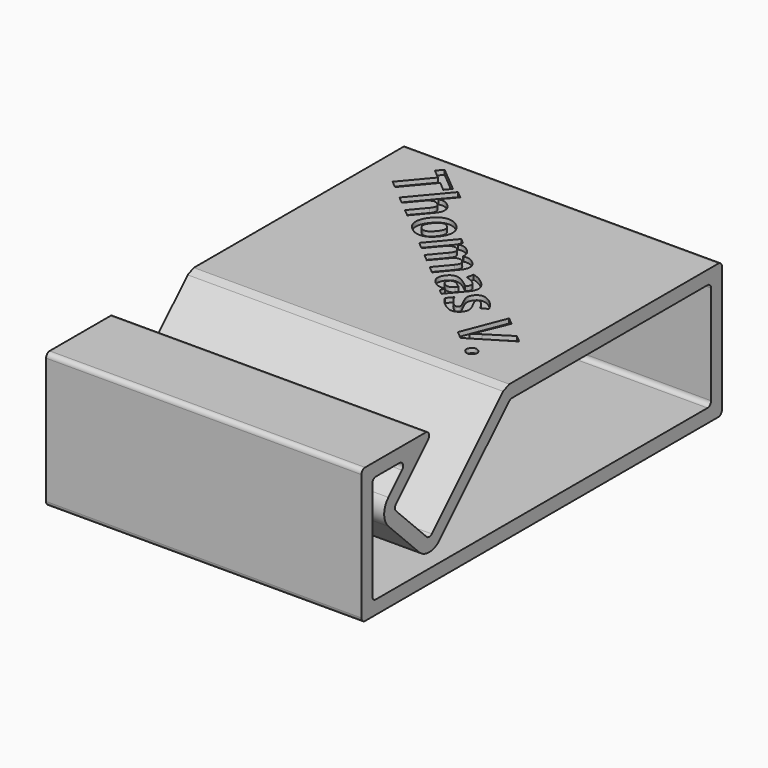
from build123d import *

# Parameters (mm, degrees)
F0_W         = 70
F0_H         = 100
F1_DEPTH     = 30
F3_DEPTH     = 146
F4_R         = 1
F5_SIZE      = 1
F6_T         = -3
F7_TEXT_SIZE = 13.6161935445
F8_DEPTH     = 1
F9_R         = 1
F10_R        = 1


# Not quite as in the source:
# - Text() gives the source's letters only with a copy of the font that has no kerning and outlines rounded to 1/6400 em; it was checked with that copy


with BuildPart() as f1:
    # F0 (on Top) → F1 (new body)
    with BuildSketch(Plane.XY):
        Rectangle(F0_W, F0_H)
    extrude(amount=F1_DEPTH)

    # F2 (on face) → F3 (cut)
    with BuildSketch(Plane.YZ.offset(35)):
        Polygon((-31.2132034356, 8.7867965644), (-10, 30), (-29.7989898732, 30), (-41.1126983722, 18.686291501), align=None)
    extrude(amount=-F3_DEPTH, mode=Mode.SUBTRACT)

    # F4
    f4_edges = [f1.edges().sort_by_distance(p)[0] for p in [
        (0, -29.79899, 30),
        (0, -41.112698, 18.686292),
        (0, -31.213203, 8.786797),
    ]]
    fillet(f4_edges, radius=F4_R)

    # F5
    f5_edges = [f1.edges().sort_by_distance(p)[0] for p in [
        (0, -10, 30),
    ]]
    chamfer(f5_edges, length=F5_SIZE)

    # F6
    f6_openings = [f1.faces().sort_by_distance(p)[0] for p in [
        (-35, 3.291092, 14.195161),
        (35, 3.291092, 14.195161),
    ]]
    offset(amount=F6_T, openings=f6_openings)

    # F7 (on face) → F8 (cut)
    with BuildSketch(Plane.XY.offset(30)):
        with Locations(Location((-30.4916797846, 39.5926552642), (0, 0, -40))):
            Text('Thomas V.', F7_TEXT_SIZE, font='Open Sans', font_style=FontStyle.BOLD, text_align=(TextAlign.LEFT, TextAlign.BOTTOM))
    extrude(amount=-F8_DEPTH, mode=Mode.SUBTRACT)

    # F9
    f9_edges = [f1.edges().sort_by_distance(p)[0] for p in [
        (0, -50, 30),
        (0, -50, 0),
        (0, 50, 0),
        (0, 50, 30),
    ]]
    fillet(f9_edges, radius=F9_R)

    # F10
    f10_edges = [f1.edges().sort_by_distance(p)[0] for p in [
        (0, 47, 27),
        (0, 47, 3),
        (0, -47, 27),
        (0, -47, 3),
        (0, -8.403263, 27),
        (0, -9.007743, 26.749616),
        (0, -37.041631, 27),
    ]]
    fillet(f10_edges, radius=F10_R)


solid = f1.part
